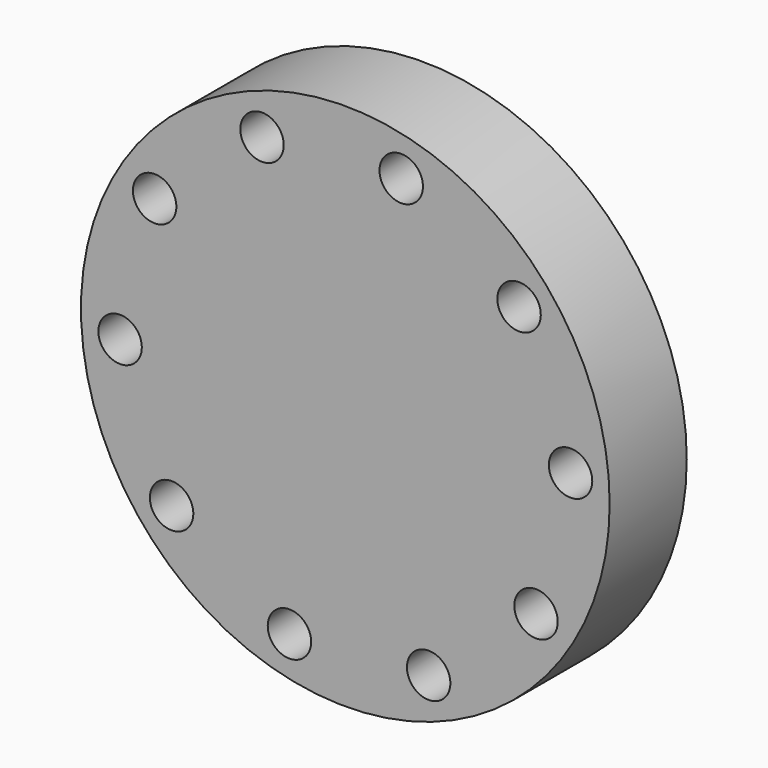
from build123d import *

# Parameters (mm, degrees)
F0_R            = 69.6849
F1_DEPTH        = 25.4
F2_R            = 5.7253497259
F3_DEPTH        = 25.401
F3_COPIES_COUNT = 10


# Not quite as in the source:
# - a pattern or mirror of a feature is missing from the dataset's text; its kind, count and spacing are read off the source's solid


with BuildPart() as f1:
    # F0 (on Front) → F1 (new body)
    with BuildSketch(Plane.XZ):
        with Locations((-61.9692653418, 36.6955287755)):
            Circle(F0_R)
    extrude(amount=F1_DEPTH)

    # F2 (on face) → F3 (cut, through all)
    with BuildSketch(Plane.XZ.offset(25.4)):
        with Locations((-83.9317291975, 91.9884815812)):
            Circle(F2_R)
    f3 = extrude(amount=-F3_DEPTH, mode=Mode.SUBTRACT)

    # F3_copies: F3 ×10 about axis
    f3_copies_axis = Axis((-61.969265, 0, 36.695529), (0, 1, 0))
    for i in range(1, F3_COPIES_COUNT):
        add(f3.rotate(f3_copies_axis, i * 360 / F3_COPIES_COUNT), mode=Mode.SUBTRACT)


solid = f1.part
